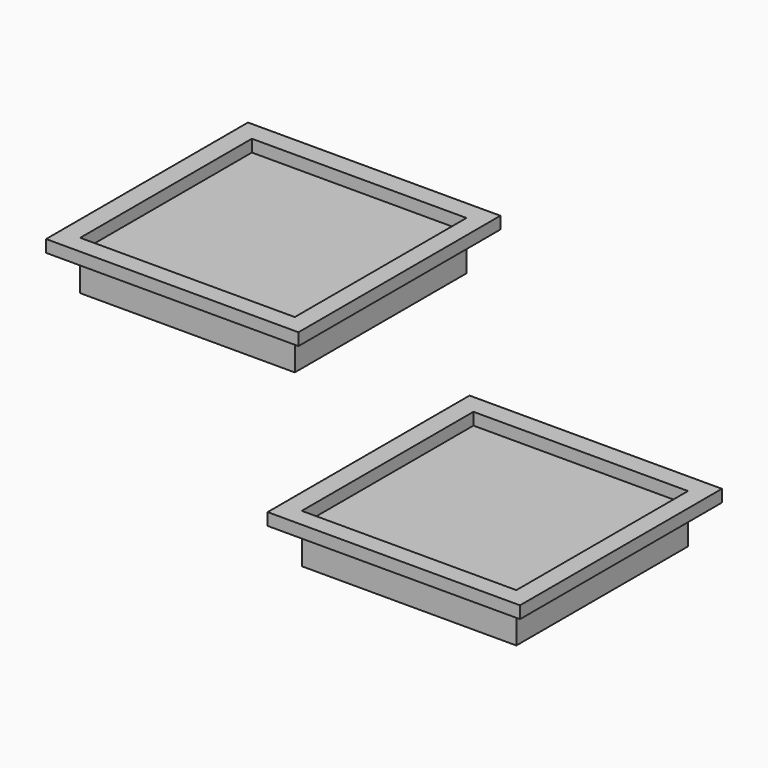
from build123d import *

# Parameters (mm, degrees)
F1_W     = 53644.8
F1_H     = 53644.8
F2_DEPTH = 9144
F1_W_2   = 63093.6
F1_H_2   = 63093.6
F3_DEPTH = 3048


# Not quite as in the source:
# - a feature names something its author has since deleted; it is built from what else it names


with BuildPart() as f2:
    # F1 (on face) → F2 (new body)
    with BuildSketch(Plane.XY):
        with Locations((-31518.0906738281, 31427.0356589794)):
            Rectangle(F1_W, F1_H)
    extrude(amount=-F2_DEPTH)


with BuildPart() as f2b:
    # F1 (on face) → F2, piece 2 (new body)
    with BuildSketch(Plane.XY):
        with Locations((74371.2, -31699.2)):
            Rectangle(F1_W, F1_H)
    extrude(amount=-F2_DEPTH)


with BuildPart() as f3:
    # F1 (on face) → F3 (new body)
    with BuildSketch(Plane.XY):
        with Locations((-31670.4906738281, 31579.4356589794)):
            Rectangle(F1_W_2, F1_H_2)
        with Locations((-31518.0906738281, 31427.0356589794)):
            Rectangle(F1_W, F1_H, mode=Mode.SUBTRACT)
    extrude(amount=F3_DEPTH)


with BuildPart() as f3b:
    # F1 (on face) → F3, piece 2 (new body)
    with BuildSketch(Plane.XY):
        with Locations((74218.8, -31546.8)):
            Rectangle(F1_W_2, F1_H_2)
        with Locations((74371.2, -31699.2)):
            Rectangle(F1_W, F1_H, mode=Mode.SUBTRACT)
    extrude(amount=F3_DEPTH)


solid = Compound([f2.part, f2b.part, f3.part, f3b.part])
